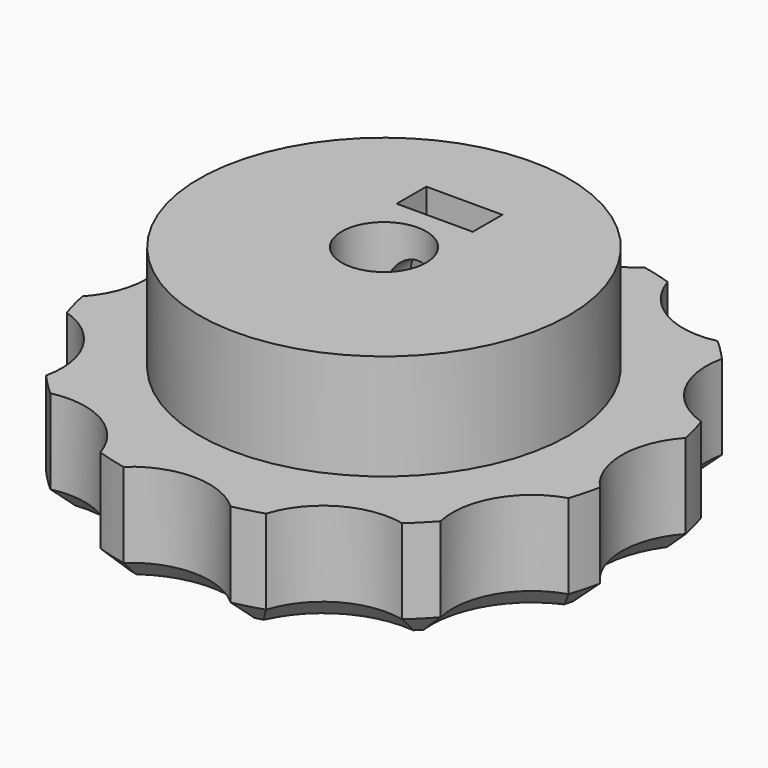
from build123d import *

# Parameters (mm, degrees)
F0_R         = 25
F1_DEPTH     = 10
F2_R         = 7.5
F3_DEPTH     = 10.001
F4_R         = 17.5
F5_DEPTH     = 10
F6_R         = 4
F7_DEPTH     = 20
F8_R         = 2.25
F9_DEPTH     = 24.4801666667
F10_W        = 7.2
F10_H        = 3.5
F11_DEPTH    = 9.2
F13_R        = 3.75
F14_DEPTH    = 13.5
F15_C1_SIZE  = 2
F15_C2_SIZE  = 2
F15_C3_SIZE  = 2
F15_C4_SIZE  = 2
F15_C5_SIZE  = 2
F15_C6_SIZE  = 2
F15_C7_SIZE  = 2
F15_C8_SIZE  = 2
F15_C9_SIZE  = 2
F15_C10_SIZE = 2
F15_C11_SIZE = 2
F15_C12_SIZE = 2
F15_C13_SIZE = 2
F15_C14_SIZE = 2
F15_C15_SIZE = 2
F15_C16_SIZE = 2
F15_C17_SIZE = 2
F15_C18_SIZE = 2
F15_C19_SIZE = 2
F15_C20_SIZE = 2
F15_C21_SIZE = 2
F15_C22_SIZE = 2
F15_C23_SIZE = 2


with BuildPart() as f1:
    # F0 (on Top) → F1 (new body)
    with BuildSketch(Plane.XY):
        Circle(F0_R)
    extrude(amount=F1_DEPTH)

    # F2 (on face) → F3 (cut, through all)
    with BuildSketch(Plane.XY.offset(10)):
        with Locations((0, 30)):
            Circle(F2_R)
        with Locations((-15, 25.9807621135)):
            Circle(F2_R)
        with Locations((-25.9807621135, 15)):
            Circle(F2_R)
        with Locations((-30, 0)):
            Circle(F2_R)
        with Locations((-25.9807621135, -15)):
            Circle(F2_R)
        with Locations((-15, -25.9807621135)):
            Circle(F2_R)
        with Locations((0, -30)):
            Circle(F2_R)
        with Locations((15, -25.9807621135)):
            Circle(F2_R)
        with Locations((25.9807621135, -15)):
            Circle(F2_R)
        with Locations((30, 0)):
            Circle(F2_R)
        with Locations((25.9807621135, 15)):
            Circle(F2_R)
        with Locations((15, 25.9807621135)):
            Circle(F2_R)
    extrude(amount=-F3_DEPTH, mode=Mode.SUBTRACT)

    # F4 (on face) → F5 (join)
    with BuildSketch(Plane.XY.offset(10)):
        Circle(F4_R)
    extrude(amount=F5_DEPTH)

    # F6 (on face) → F7 (cut, through all)
    with BuildSketch(Plane.XY.offset(20)):
        Circle(F6_R)
    extrude(amount=-F7_DEPTH, mode=Mode.SUBTRACT)

    # F8 (on Front) → F9 (cut, through all)
    with BuildSketch(Plane.XZ):
        with Locations((0, 15)):
            Circle(F8_R)
    extrude(amount=-F9_DEPTH, mode=Mode.SUBTRACT)

    # F10 (on face) → F11 (cut)
    with BuildSketch(Plane.XY.offset(20)):
        with Locations((0, 7.75)):
            Rectangle(F10_W, F10_H)
    extrude(amount=-F11_DEPTH, mode=Mode.SUBTRACT)

    # F13 (on offset) → F14 (cut, through all)
    with BuildSketch(Plane.XZ.offset(-25)):
        with Locations((0, 15)):
            Circle(F13_R)
    extrude(amount=F14_DEPTH, mode=Mode.SUBTRACT)

    # F15: chamfer of 2 on 23 edges, made by hand

    # F15_c1
    f15_c1_edges = [f1.edges().sort_by_distance(p)[0] for p in [
        (24.1481456572, 6.4704761276, 0),
    ]]
    chamfer(f15_c1_edges, length=F15_C1_SIZE)

    # F15_c2
    f15_c2_edges = [f1.edges().sort_by_distance(p)[0] for p in [
        (22.6680317958, -1.5786837087, 0),
    ]]
    chamfer(f15_c2_edges, length=F15_C2_SIZE)

    # F15_c3
    f15_c3_edges = [f1.edges().sort_by_distance(p)[0] for p in [
        (23.8267406055, -7.5687800944, 0),
    ]]
    chamfer(f15_c3_edges, length=F15_C3_SIZE)

    # F15_c4
    f15_c4_edges = [f1.edges().sort_by_distance(p)[0] for p in [
        (18.8417495346, 12.7011960942, 0),
    ]]
    chamfer(f15_c4_edges, length=F15_C4_SIZE)

    # F15_c5
    f15_c5_edges = [f1.edges().sort_by_distance(p)[0] for p in [
        (18.8417495346, -12.7011960942, 0),
    ]]
    chamfer(f15_c5_edges, length=F15_C5_SIZE)

    # F15_c6
    f15_c6_edges = [f1.edges().sort_by_distance(p)[0] for p in [
        (16.8501726066, 18.4681261401, 0),
    ]]
    chamfer(f15_c6_edges, length=F15_C6_SIZE)

    # F15_c7
    f15_c7_edges = [f1.edges().sort_by_distance(p)[0] for p in [
        (16.8501726066, -18.4681261401, 0),
    ]]
    chamfer(f15_c7_edges, length=F15_C7_SIZE)

    # F15_c8
    f15_c8_edges = [f1.edges().sort_by_distance(p)[0] for p in [
        (9.9668357016, 20.4204332433, 0),
    ]]
    chamfer(f15_c8_edges, length=F15_C8_SIZE)

    # F15_c9
    f15_c9_edges = [f1.edges().sort_by_distance(p)[0] for p in [
        (9.9668357016, -20.4204332433, 0),
    ]]
    chamfer(f15_c9_edges, length=F15_C9_SIZE)

    # F15_c10
    f15_c10_edges = [f1.edges().sort_by_distance(p)[0] for p in [
        (5.3586144654, 24.418952701, 0),
    ]]
    chamfer(f15_c10_edges, length=F15_C10_SIZE)

    # F15_c11
    f15_c11_edges = [f1.edges().sort_by_distance(p)[0] for p in [
        (5.3586144654, -24.418952701, 0),
    ]]
    chamfer(f15_c11_edges, length=F15_C11_SIZE)

    # F15_c12
    f15_c12_edges = [f1.edges().sort_by_distance(p)[0] for p in [
        (-1.5786837087, 22.6680317958, 0),
    ]]
    chamfer(f15_c12_edges, length=F15_C12_SIZE)

    # F15_c13
    f15_c13_edges = [f1.edges().sort_by_distance(p)[0] for p in [
        (-1.5786837087, -22.6680317958, 0),
    ]]
    chamfer(f15_c13_edges, length=F15_C13_SIZE)

    # F15_c14
    f15_c14_edges = [f1.edges().sort_by_distance(p)[0] for p in [
        (-7.5687800944, 23.8267406055, 0),
    ]]
    chamfer(f15_c14_edges, length=F15_C14_SIZE)

    # F15_c15
    f15_c15_edges = [f1.edges().sort_by_distance(p)[0] for p in [
        (-7.5687800944, -23.8267406055, 0),
    ]]
    chamfer(f15_c15_edges, length=F15_C15_SIZE)

    # F15_c16
    f15_c16_edges = [f1.edges().sort_by_distance(p)[0] for p in [
        (-12.7011960942, 18.8417495346, 0),
    ]]
    chamfer(f15_c16_edges, length=F15_C16_SIZE)

    # F15_c17
    f15_c17_edges = [f1.edges().sort_by_distance(p)[0] for p in [
        (-12.7011960942, -18.8417495346, 0),
    ]]
    chamfer(f15_c17_edges, length=F15_C17_SIZE)

    # F15_c18
    f15_c18_edges = [f1.edges().sort_by_distance(p)[0] for p in [
        (-18.4681261401, 16.8501726066, 0),
    ]]
    chamfer(f15_c18_edges, length=F15_C18_SIZE)

    # F15_c19
    f15_c19_edges = [f1.edges().sort_by_distance(p)[0] for p in [
        (-18.4681261401, -16.8501726066, 0),
    ]]
    chamfer(f15_c19_edges, length=F15_C19_SIZE)

    # F15_c20
    f15_c20_edges = [f1.edges().sort_by_distance(p)[0] for p in [
        (-20.4204332433, 9.9668357016, 0),
    ]]
    chamfer(f15_c20_edges, length=F15_C20_SIZE)

    # F15_c21
    f15_c21_edges = [f1.edges().sort_by_distance(p)[0] for p in [
        (-20.4204332433, -9.9668357016, 0),
    ]]
    chamfer(f15_c21_edges, length=F15_C21_SIZE)

    # F15_c22
    f15_c22_edges = [f1.edges().sort_by_distance(p)[0] for p in [
        (-24.418952701, -5.3586144654, 0),
    ]]
    chamfer(f15_c22_edges, length=F15_C22_SIZE)

    # F15_c23
    f15_c23_edges = [f1.edges().sort_by_distance(p)[0] for p in [
        (-22.6680317958, 1.5786837087, 0),
    ]]
    chamfer(f15_c23_edges, length=F15_C23_SIZE)


solid = f1.part
